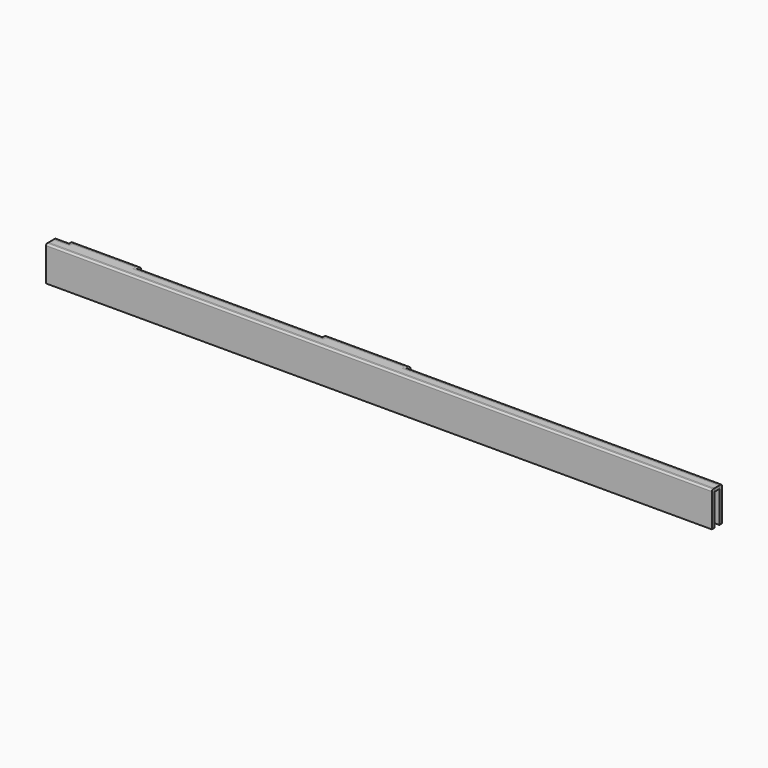
from build123d import *

# Parameters (mm, degrees)
F0_W     = 20
F0_H     = 1
F0_W_2   = 25
F1_DEPTH = 1
F2_DEPTH = 11
F0_W_3   = 210
F3_R     = 0.5
F3_2_R   = 0.5


with BuildPart() as f1:
    # F0 (on Top) → F1 (new body)
    with BuildSketch(Plane.XY):
        Polygon((-100, -6), (-105, -6), (-105, -8), (105, -8), (105, -6), (5, -6), (-20, -6), (-80, -6), align=None)
        with Locations((-90, -5.5)):
            Rectangle(F0_W, F0_H)
        with Locations((-7.5, -5.5)):
            Rectangle(F0_W_2, F0_H)
    extrude(amount=-F1_DEPTH)


with BuildPart() as f2:
    # F0 (on Top) → F2 (new body)
    with BuildSketch(Plane.XY):
        Polygon((-101, -4), (-101, -5), (-100, -5), (-80, -5), (-79, -5), (-79, -4), align=None)
        Polygon((-101, -5), (-105, -5), (-105, -6), (-100, -6), (-100, -5), align=None)
        Polygon((-79, -5), (-80, -5), (-80, -6), (-20, -6), (-20, -5), (-21, -5), align=None)
        Polygon((-21, -4), (-21, -5), (-20, -5), (5, -5), (6, -5), (6, -4), align=None)
        Polygon((5, -6), (105, -6), (105, -5), (6, -5), (5, -5), align=None)
    extrude(amount=-F2_DEPTH)

    # F3
    f3_edges = [f2.edges().sort_by_distance(p)[0] for p in [
        (-103, -5, 0),
        (-21, -4.5, 0),
        (-7.5, -4, 0),
        (6, -4.5, 0),
        (55.5, -5, 0),
        (-90, -4, 0),
        (-79, -4.5, 0),
        (-101, -4.5, 0),
        (-50, -5, 0),
    ]]
    fillet(f3_edges, radius=F3_R)


with BuildPart() as f2b:
    # F0 (on Top) → F2, piece 2 (new body)
    with BuildSketch(Plane.XY):
        with Locations((0, -8.5)):
            Rectangle(F0_W_3, F0_H)
    extrude(amount=-F2_DEPTH)

    # F3#2
    f3_2_edges = [f2b.edges().sort_by_distance(p)[0] for p in [
        (0, -9, 0),
    ]]
    fillet(f3_2_edges, radius=F3_2_R)


solid = Compound([f1.part, f2.part, f2b.part])
